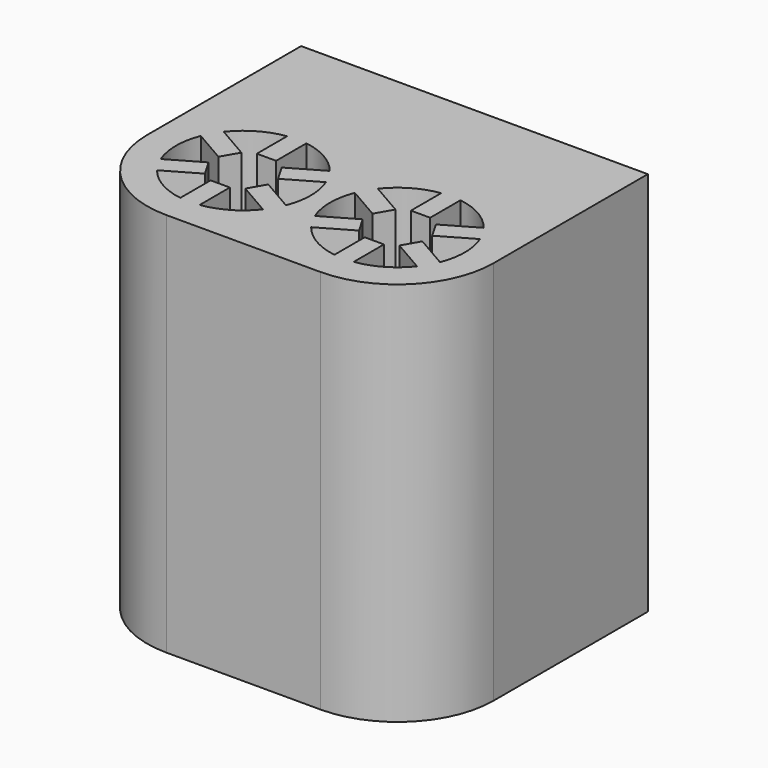
from build123d import *

# Parameters (mm, degrees)
F1_DEPTH = 10
F2_R     = 1.4
F3_DEPTH = 4


# Not quite as in the source:
# - a feature names something its author has since deleted; it is built from what else it names


with BuildPart() as f1:
    # F0 (on Top) → F1 (new body, symmetric)
    with BuildSketch(Plane.XY):
        with BuildLine():
            ThreePointArc((0, -5), (3.5355339059, -3.5355339059), (5, 0))
            Line((5, 0), (5, 10))
            Line((5, 10), (-13, 10))
            Line((-13, 10), (-13, 0))
            ThreePointArc((-13, 0), (-11.5355339059, -3.5355339059), (-8, -5))
            Line((-8, -5), (0, -5))
        make_face()
        with BuildLine():
            ThreePointArc((-10.75, 2.1650635095), (-9.75, 3.0310889132), (-8.5, 3.4641016151))
            ThreePointArc((-8.5, 3.4641016151), (-8, 3.5), (-7.5, 3.4641016151))
            ThreePointArc((-7.5, 3.4641016151), (-6.25, 3.0310889132), (-5.25, 2.1650635095))
            Line((-5.25, 2.1650635095), (-6.9509618943, 1.1830127019))
            Line((-6.9509618943, 1.1830127019), (-6.4509618943, 0.3169872981))
            Line((-6.4509618943, 0.3169872981), (-4.75, 1.2990381057))
            ThreePointArc((-4.75, 1.2990381057), (-4.5, 0), (-4.75, -1.2990381057))
            Line((-4.75, -1.2990381057), (-6.4509618943, -0.3169872981))
            Line((-6.4509618943, -0.3169872981), (-6.9509618943, -1.1830127019))
            Line((-6.9509618943, -1.1830127019), (-5.25, -2.1650635095))
            ThreePointArc((-5.25, -2.1650635095), (-6.25, -3.0310889132), (-7.5, -3.4641016151))
            Line((-7.5, -3.4641016151), (-7.5, -1.5))
            Line((-7.5, -1.5), (-8.5, -1.5))
            Line((-8.5, -1.5), (-8.5, -3.4641016151))
            ThreePointArc((-8.5, -3.4641016151), (-9.75, -3.0310889132), (-10.75, -2.1650635095))
            Line((-10.75, -2.1650635095), (-9.0490381057, -1.1830127019))
            Line((-9.0490381057, -1.1830127019), (-9.5490381057, -0.3169872981))
            Line((-9.5490381057, -0.3169872981), (-11.25, -1.2990381057))
            ThreePointArc((-11.25, -1.2990381057), (-11.5, 0), (-11.25, 1.2990381057))
            Line((-11.25, 1.2990381057), (-9.5490381057, 0.3169872981))
            Line((-9.5490381057, 0.3169872981), (-9.0490381057, 1.1830127019))
            Line((-9.0490381057, 1.1830127019), (-10.75, 2.1650635095))
        make_face(mode=Mode.SUBTRACT)
        with BuildLine():
            ThreePointArc((-2.75, 2.1650635095), (-1.75, 3.0310889132), (-0.5, 3.4641016151))
            ThreePointArc((-0.5, 3.4641016151), (0, 3.5), (0.5, 3.4641016151))
            ThreePointArc((0.5, 3.4641016151), (1.75, 3.0310889132), (2.75, 2.1650635095))
            Line((2.75, 2.1650635095), (1.0490381057, 1.1830127019))
            Line((1.0490381057, 1.1830127019), (1.5490381057, 0.3169872981))
            Line((1.5490381057, 0.3169872981), (3.25, 1.2990381057))
            ThreePointArc((3.25, 1.2990381057), (3.5, 0), (3.25, -1.2990381057))
            Line((3.25, -1.2990381057), (1.5490381057, -0.3169872981))
            Line((1.5490381057, -0.3169872981), (1.0490381057, -1.1830127019))
            Line((1.0490381057, -1.1830127019), (2.75, -2.1650635095))
            ThreePointArc((2.75, -2.1650635095), (1.75, -3.0310889132), (0.5, -3.4641016151))
            Line((0.5, -3.4641016151), (0.5, -1.5))
            Line((0.5, -1.5), (-0.5, -1.5))
            Line((-0.5, -1.5), (-0.5, -3.4641016151))
            ThreePointArc((-0.5, -3.4641016151), (-1.75, -3.0310889132), (-2.75, -2.1650635095))
            Line((-2.75, -2.1650635095), (-1.0490381057, -1.1830127019))
            Line((-1.0490381057, -1.1830127019), (-1.5490381057, -0.3169872981))
            Line((-1.5490381057, -0.3169872981), (-3.25, -1.2990381057))
            ThreePointArc((-3.25, -1.2990381057), (-3.5, 0), (-3.25, 1.2990381057))
            Line((-3.25, 1.2990381057), (-1.5490381057, 0.3169872981))
            Line((-1.5490381057, 0.3169872981), (-1.0490381057, 1.1830127019))
            Line((-1.0490381057, 1.1830127019), (-2.75, 2.1650635095))
        make_face(mode=Mode.SUBTRACT)
        with BuildLine():
            ThreePointArc((0.5, 3.4641016151), (0, 3.5), (-0.5, 3.4641016151))
            Line((-0.5, 3.4641016151), (-0.5, 1.5))
            Line((-0.5, 1.5), (0.5, 1.5))
            Line((0.5, 1.5), (0.5, 3.4641016151))
        make_face()
        with BuildLine():
            ThreePointArc((-7.5, 3.4641016151), (-8, 3.5), (-8.5, 3.4641016151))
            Line((-8.5, 3.4641016151), (-8.5, 1.5))
            Line((-8.5, 1.5), (-7.5, 1.5))
            Line((-7.5, 1.5), (-7.5, 3.4641016151))
        make_face()
    extrude(amount=F1_DEPTH, both=True)

    # F2 (on face) → F3 (cut)
    with BuildSketch(Plane(origin=(-13, 0, 0), x_dir=(0, -1, 0), z_dir=(-1, 0, 0))):
        with Locations((-7.5, -4)):
            Circle(F2_R)
    extrude(amount=-F3_DEPTH, mode=Mode.SUBTRACT)


solid = f1.part
